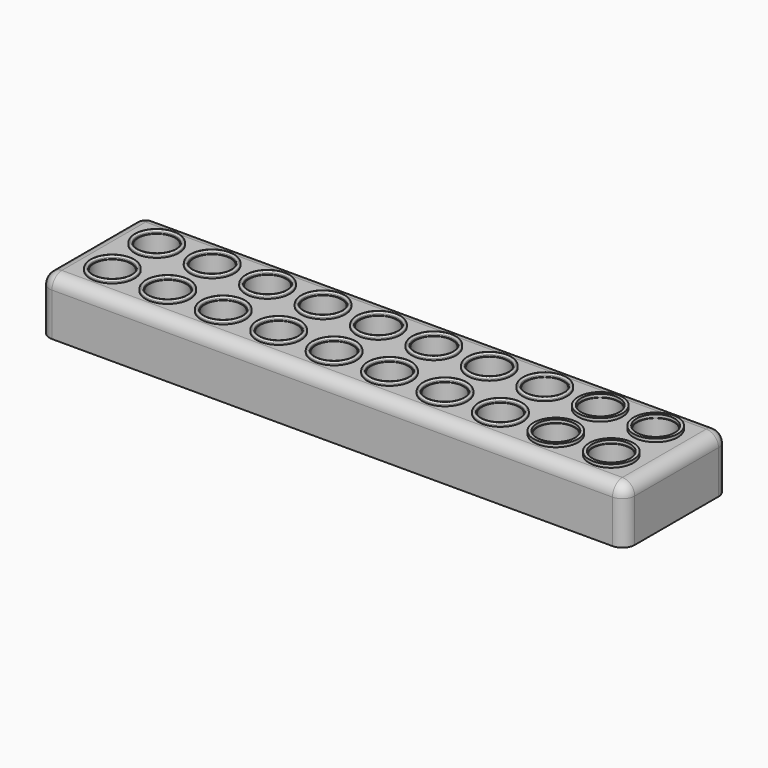
from build123d import *

# Parameters (mm, degrees)
F0_W     = 190
F0_H     = 42
F0_R     = 6
F1_DEPTH = 16
F2_DEPTH = 2
F3_R     = 4
F4_R     = 7.2
F4_R_2   = 6.2
F5_DEPTH = 1
F6_R     = 0.49999


# Not quite as in the source:
# - a fillet or chamfer is up to 0.001 mm smaller than in the source, because OpenCascade refuses the exact size
# - a feature names something its author has since deleted; it is built from what else it names


with BuildPart() as f1:
    # F0 (on Top) → F1 (new body)
    with BuildSketch(Plane.XY):
        with Locations((67.449604854, 20.0262753442)):
            Rectangle(F0_W, F0_H)
        with Locations((-13.550395146, 11.0262753442)):
            Circle(F0_R, mode=Mode.SUBTRACT)
        with Locations((4.449604854, 11.0262753442)):
            Circle(F0_R, mode=Mode.SUBTRACT)
        with Locations((22.449604854, 11.0262753442)):
            Circle(F0_R, mode=Mode.SUBTRACT)
        with Locations((40.449604854, 11.0262753442)):
            Circle(F0_R, mode=Mode.SUBTRACT)
        with Locations((58.449604854, 11.0262753442)):
            Circle(F0_R, mode=Mode.SUBTRACT)
        with Locations((76.449604854, 11.0262753442)):
            Circle(F0_R, mode=Mode.SUBTRACT)
        with Locations((94.449604854, 11.0262753442)):
            Circle(F0_R, mode=Mode.SUBTRACT)
        with Locations((112.449604854, 11.0262753442)):
            Circle(F0_R, mode=Mode.SUBTRACT)
        with Locations((130.449604854, 11.0262753442)):
            Circle(F0_R, mode=Mode.SUBTRACT)
        with Locations((148.449604854, 11.0262753442)):
            Circle(F0_R, mode=Mode.SUBTRACT)
        with Locations((-13.550395146, 29.0262753442)):
            Circle(F0_R, mode=Mode.SUBTRACT)
        with Locations((4.449604854, 29.0262753442)):
            Circle(F0_R, mode=Mode.SUBTRACT)
        with Locations((22.449604854, 29.0262753442)):
            Circle(F0_R, mode=Mode.SUBTRACT)
        with Locations((40.449604854, 29.0262753442)):
            Circle(F0_R, mode=Mode.SUBTRACT)
        with Locations((58.449604854, 29.0262753442)):
            Circle(F0_R, mode=Mode.SUBTRACT)
        with Locations((76.449604854, 29.0262753442)):
            Circle(F0_R, mode=Mode.SUBTRACT)
        with Locations((94.449604854, 29.0262753442)):
            Circle(F0_R, mode=Mode.SUBTRACT)
        with Locations((112.449604854, 29.0262753442)):
            Circle(F0_R, mode=Mode.SUBTRACT)
        with Locations((130.449604854, 29.0262753442)):
            Circle(F0_R, mode=Mode.SUBTRACT)
        with Locations((148.449604854, 29.0262753442)):
            Circle(F0_R, mode=Mode.SUBTRACT)
    extrude(amount=F1_DEPTH)

    # F0 (on Top) → F2 (join)
    with BuildSketch(Plane.XY):
        with Locations((67.449604854, 20.0262753442)):
            Rectangle(F0_W, F0_H)
        with Locations((-13.550395146, 11.0262753442)):
            Circle(F0_R, mode=Mode.SUBTRACT)
        with Locations((4.449604854, 11.0262753442)):
            Circle(F0_R, mode=Mode.SUBTRACT)
        with Locations((22.449604854, 11.0262753442)):
            Circle(F0_R, mode=Mode.SUBTRACT)
        with Locations((40.449604854, 11.0262753442)):
            Circle(F0_R, mode=Mode.SUBTRACT)
        with Locations((58.449604854, 11.0262753442)):
            Circle(F0_R, mode=Mode.SUBTRACT)
        with Locations((76.449604854, 11.0262753442)):
            Circle(F0_R, mode=Mode.SUBTRACT)
        with Locations((94.449604854, 11.0262753442)):
            Circle(F0_R, mode=Mode.SUBTRACT)
        with Locations((112.449604854, 11.0262753442)):
            Circle(F0_R, mode=Mode.SUBTRACT)
        with Locations((130.449604854, 11.0262753442)):
            Circle(F0_R, mode=Mode.SUBTRACT)
        with Locations((148.449604854, 11.0262753442)):
            Circle(F0_R, mode=Mode.SUBTRACT)
        with Locations((-13.550395146, 29.0262753442)):
            Circle(F0_R, mode=Mode.SUBTRACT)
        with Locations((4.449604854, 29.0262753442)):
            Circle(F0_R, mode=Mode.SUBTRACT)
        with Locations((22.449604854, 29.0262753442)):
            Circle(F0_R, mode=Mode.SUBTRACT)
        with Locations((40.449604854, 29.0262753442)):
            Circle(F0_R, mode=Mode.SUBTRACT)
        with Locations((58.449604854, 29.0262753442)):
            Circle(F0_R, mode=Mode.SUBTRACT)
        with Locations((76.449604854, 29.0262753442)):
            Circle(F0_R, mode=Mode.SUBTRACT)
        with Locations((94.449604854, 29.0262753442)):
            Circle(F0_R, mode=Mode.SUBTRACT)
        with Locations((112.449604854, 29.0262753442)):
            Circle(F0_R, mode=Mode.SUBTRACT)
        with Locations((130.449604854, 29.0262753442)):
            Circle(F0_R, mode=Mode.SUBTRACT)
        with Locations((148.449604854, 29.0262753442)):
            Circle(F0_R, mode=Mode.SUBTRACT)
        with Locations((-13.550395146, 29.0262753442)):
            Circle(F0_R)
        with Locations((-13.550395146, 11.0262753442)):
            Circle(F0_R)
        with Locations((4.449604854, 11.0262753442)):
            Circle(F0_R)
        with Locations((4.449604854, 29.0262753442)):
            Circle(F0_R)
        with Locations((22.449604854, 29.0262753442)):
            Circle(F0_R)
        with Locations((22.449604854, 11.0262753442)):
            Circle(F0_R)
        with Locations((40.449604854, 29.0262753442)):
            Circle(F0_R)
        with Locations((40.449604854, 11.0262753442)):
            Circle(F0_R)
        with Locations((58.449604854, 11.0262753442)):
            Circle(F0_R)
        with Locations((58.449604854, 29.0262753442)):
            Circle(F0_R)
        with Locations((76.449604854, 29.0262753442)):
            Circle(F0_R)
        with Locations((76.449604854, 11.0262753442)):
            Circle(F0_R)
        with Locations((94.449604854, 11.0262753442)):
            Circle(F0_R)
        with Locations((94.449604854, 29.0262753442)):
            Circle(F0_R)
        with Locations((112.449604854, 29.0262753442)):
            Circle(F0_R)
        with Locations((112.449604854, 11.0262753442)):
            Circle(F0_R)
        with Locations((130.449604854, 29.0262753442)):
            Circle(F0_R)
        with Locations((130.449604854, 11.0262753442)):
            Circle(F0_R)
        with Locations((148.449604854, 11.0262753442)):
            Circle(F0_R)
        with Locations((148.449604854, 29.0262753442)):
            Circle(F0_R)
    extrude(amount=-F2_DEPTH)

    # F3
    f3_edges = [f1.edges().sort_by_distance(p)[0] for p in [
        (67.449605, -0.973725, 16),
        (162.449605, 20.026275, 16),
        (67.449605, 41.026275, 16),
        (-27.550395, 20.026275, 16),
        (-27.550395, 41.026275, 7),
        (162.449605, 41.026275, 7),
        (-27.550395, -0.973725, 7),
        (162.449605, -0.973725, 7),
    ]]
    fillet(f3_edges, radius=F3_R)

    # F4 (on face) → F5 (join)
    with BuildSketch(Plane.XY.offset(16)):
        with Locations((-13.550395146, 11.0262753442)):
            Circle(F4_R)
        with Locations((-13.550395146, 11.0262753442)):
            Circle(F4_R_2, mode=Mode.SUBTRACT)
        with Locations((-13.550395146, 29.0262753442)):
            Circle(F4_R)
        with Locations((-13.550395146, 29.0262753442)):
            Circle(F4_R_2, mode=Mode.SUBTRACT)
        with Locations((4.449604854, 29.0262753442)):
            Circle(F4_R)
        with Locations((4.449604854, 29.0262753442)):
            Circle(F4_R_2, mode=Mode.SUBTRACT)
        with Locations((4.449604854, 11.0262753442)):
            Circle(F4_R)
        with Locations((4.449604854, 11.0262753442)):
            Circle(F4_R_2, mode=Mode.SUBTRACT)
        with Locations((22.449604854, 29.0262753442)):
            Circle(F4_R)
        with Locations((22.449604854, 29.0262753442)):
            Circle(F4_R_2, mode=Mode.SUBTRACT)
        with Locations((22.449604854, 11.0262753442)):
            Circle(F4_R)
        with Locations((22.449604854, 11.0262753442)):
            Circle(F4_R_2, mode=Mode.SUBTRACT)
        with Locations((40.449604854, 11.0262753442)):
            Circle(F4_R)
        with Locations((40.449604854, 11.0262753442)):
            Circle(F4_R_2, mode=Mode.SUBTRACT)
        with Locations((40.449604854, 29.0262753442)):
            Circle(F4_R)
        with Locations((40.449604854, 29.0262753442)):
            Circle(F4_R_2, mode=Mode.SUBTRACT)
        with Locations((58.449604854, 11.0262753442)):
            Circle(F4_R)
        with Locations((58.449604854, 11.0262753442)):
            Circle(F4_R_2, mode=Mode.SUBTRACT)
        with Locations((58.449604854, 29.0262753442)):
            Circle(F4_R)
        with Locations((58.449604854, 29.0262753442)):
            Circle(F4_R_2, mode=Mode.SUBTRACT)
        with Locations((76.449604854, 29.0262753442)):
            Circle(F4_R)
        with Locations((76.449604854, 29.0262753442)):
            Circle(F4_R_2, mode=Mode.SUBTRACT)
        with Locations((76.449604854, 11.0262753442)):
            Circle(F4_R)
        with Locations((76.449604854, 11.0262753442)):
            Circle(F4_R_2, mode=Mode.SUBTRACT)
        with Locations((94.449604854, 11.0262753442)):
            Circle(F4_R)
        with Locations((94.449604854, 11.0262753442)):
            Circle(F4_R_2, mode=Mode.SUBTRACT)
        with Locations((112.449604854, 11.0262753442)):
            Circle(F4_R)
        with Locations((112.449604854, 11.0262753442)):
            Circle(F4_R_2, mode=Mode.SUBTRACT)
        with Locations((112.449604854, 29.0262753442)):
            Circle(F4_R)
        with Locations((112.449604854, 29.0262753442)):
            Circle(F4_R_2, mode=Mode.SUBTRACT)
        with Locations((94.449604854, 29.0262753442)):
            Circle(F4_R)
        with Locations((94.449604854, 29.0262753442)):
            Circle(F4_R_2, mode=Mode.SUBTRACT)
        with Locations((130.449604854, 29.0262753442)):
            Circle(F4_R)
        with Locations((130.449604854, 29.0262753442)):
            Circle(F4_R_2, mode=Mode.SUBTRACT)
        with Locations((130.449604854, 11.0262753442)):
            Circle(F4_R)
        with Locations((130.449604854, 11.0262753442)):
            Circle(F4_R_2, mode=Mode.SUBTRACT)
        with Locations((148.449604854, 11.0262753442)):
            Circle(F4_R)
        with Locations((148.449604854, 11.0262753442)):
            Circle(F4_R_2, mode=Mode.SUBTRACT)
        with Locations((148.449604854, 29.0262753442)):
            Circle(F4_R)
        with Locations((148.449604854, 29.0262753442)):
            Circle(F4_R_2, mode=Mode.SUBTRACT)
    extrude(amount=F5_DEPTH)

    # F6 (radius 0.5 in the source; OpenCascade refuses exactly that, so slightly less here)
    f6_edges = [f1.edges().sort_by_distance(p)[0] for p in [
        (-20.750395, 11.026275, 17),
        (-19.750395, 11.026275, 17),
        (-2.750395, 11.026275, 17),
        (-1.750395, 11.026275, 17),
        (-2.750395, 29.026275, 17),
        (-1.750395, 29.026275, 17),
        (-20.750395, 29.026275, 17),
        (-19.750395, 29.026275, 17),
        (15.249605, 29.026275, 17),
        (16.249605, 29.026275, 17),
        (15.249605, 11.026275, 17),
        (16.249605, 11.026275, 17),
        (51.249605, 11.026275, 17),
        (52.249605, 11.026275, 17),
        (69.249605, 29.026275, 17),
        (70.249605, 29.026275, 17),
        (51.249605, 29.026275, 17),
        (52.249605, 29.026275, 17),
        (87.249605, 29.026275, 17),
        (88.249605, 29.026275, 17),
        (87.249605, 11.026275, 17),
        (88.249605, 11.026275, 17),
        (105.249605, 11.026275, 17),
        (106.249605, 11.026275, 17),
        (105.249605, 29.026275, 17),
        (106.249605, 29.026275, 17),
        (33.249605, 11.026275, 17),
        (34.249605, 11.026275, 17),
        (33.249605, 29.026275, 17),
        (34.249605, 29.026275, 17),
        (69.249605, 11.026275, 17),
        (70.249605, 11.026275, 17),
    ]]
    fillet(f6_edges, radius=F6_R)


solid = f1.part
